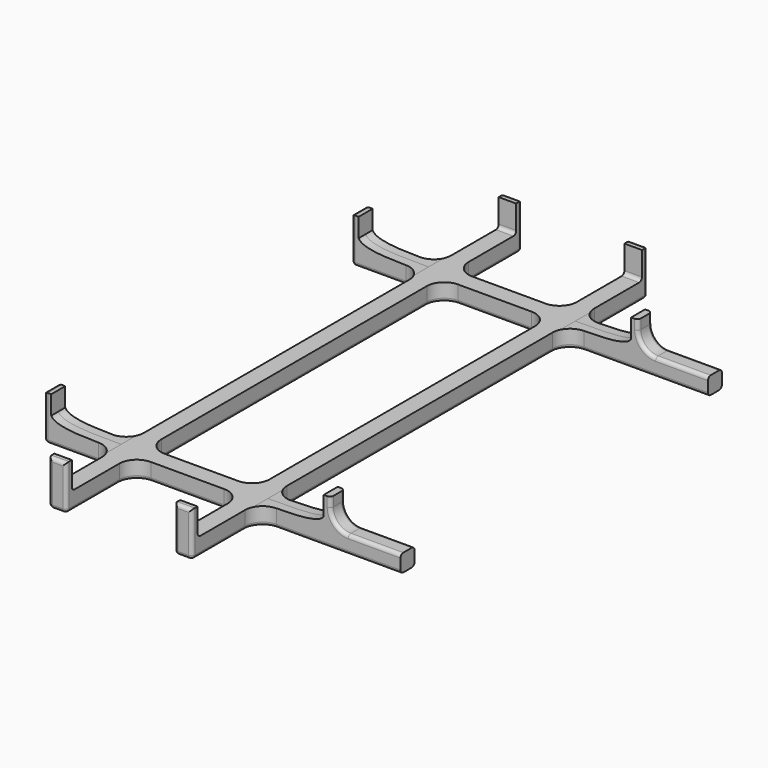
from build123d import *

# Parameters (mm, degrees)
F1_DEPTH  = 2.5
F3_DEPTH  = 2.5
F9_W      = 5
F9_H      = 5
F10_DEPTH = 20
F11_W     = 5
F11_H     = 5
F12_DEPTH = 20
F13_R     = 5
F14_R     = 1


with BuildPart() as f1:
    # F0 (on Front) → F1 (new body, symmetric)
    with BuildSketch(Plane.XZ):
        Polygon((-39, 7.8), (-41, 7.8), (-41, -5), (41, -5), (41, 7.8), (39, 7.8), (39, 2.4), (39, 0), (21, 0), (-21, 0), (-39, 0), (-39, 2.4), align=None)
        with BuildLine():
            Line((-39, 0), (-21, 0))
            add(Edge.make_bspline(
                [(-39, 2.4), (-37.8, 0), (-30, 0), (-21, 0)],
                knots=[0, 0, 0, 0, 18.1592951405, 18.1592951405, 18.1592951405, 18.1592951405], degree=3))
            Line((-39, 2.4), (-39, 0))
        make_face()
        with BuildLine():
            add(Edge.make_bspline(
                [(39, 2.4), (37.8, 0), (30, 0), (21, 0)],
                knots=[0, 0, 0, 0, 18.1592951405, 18.1592951405, 18.1592951405, 18.1592951405], degree=3))
            Line((21, 0), (39, 0))
            Line((39, 0), (39, 2.4))
        make_face()
    extrude(amount=F1_DEPTH, both=True)


with BuildPart() as f3:
    # F2 (on Right) → F3 (new body, symmetric)
    with BuildSketch(Plane.YZ):
        Polygon((-79.5, 7.8), (-81.5, 7.8), (-81.5, -5), (81.5, -5), (81.5, 7.8), (79.5, 7.8), (79.5, 0), (-79.5, 0), align=None)
    extrude(amount=F3_DEPTH, both=True)


with BuildPart() as f1_1:
    # F4: moved
    add(f1.part.moved(Location((0, -55, 0))))


with BuildPart() as f5_1:
    # F5: copy of F1
    add(f1_1.part.moved(Location((0, 110, 0))))


with BuildPart() as f3_1:
    # F6: moved
    add(f3.part.moved(Location((-18, 0, 0))))


with BuildPart() as f7_1:
    # F7: copy of F3
    add(f3_1.part.moved(Location((36, 0, 0))))


with BuildPart() as f1_2:
    add(f1_1.part)

    # F8: union F3, F7_1, F5_1
    add(f3_1.part)
    add(f7_1.part)
    add(f5_1.part)

    # F9 (on face) → F10 (join)
    with BuildSketch(Plane.YZ.offset(41)):
        with Locations((-55, -2.5)):
            Rectangle(F9_W, F9_H)
    extrude(amount=F10_DEPTH)

    # F11 (on face) → F12 (join)
    with BuildSketch(Plane.YZ.offset(41)):
        with Locations((55, -2.5)):
            Rectangle(F11_W, F11_H)
    extrude(amount=F12_DEPTH)

    # F13
    f13_edges = [f1_2.edges().sort_by_distance(p)[0] for p in [
        (-15.5, 52.5, -2.5),
        (-15.5, 57.5, -2.5),
        (-20.5, 52.5, -2.5),
        (-20.5, 57.5, -2.5),
        (15.5, 57.5, -2.5),
        (15.5, 52.5, -2.5),
        (20.5, 57.5, -2.5),
        (20.5, 52.5, -2.5),
        (20.5, -57.5, -2.5),
        (20.5, -52.5, -2.5),
        (15.5, -52.5, -2.5),
        (15.5, -57.5, -2.5),
        (-20.5, -57.5, -2.5),
        (-15.5, -57.5, -2.5),
        (-15.5, -52.5, -2.5),
        (-20.5, -52.5, -2.5),
        (41, -55, 0),
        (41, 55, 0),
    ]]
    fillet(f13_edges, radius=F13_R)

    # F14
    f14_edges = [f1_2.edges().sort_by_distance(p)[0] for p in [
        (53.5, 52.5, 0),
        (53.5, 57.5, 0),
        (53.5, -57.5, 0),
        (53.5, -52.5, 0),
        (43.25, -57.5, -5),
        (43.25, -52.5, -5),
        (43.25, 57.5, -5),
        (18, 81.5, -5),
        (15.5, 72, -5),
        (-18, 81.5, -5),
        (-20.5, 72, -5),
        (-41, 55, -5),
        (-33.25, 52.5, -5),
        (-41, -55, -5),
        (-33.25, -57.5, -5),
        (-18, -81.5, -5),
        (-15.5, -72, -5),
        (18, -81.5, -5),
        (-15.5, 0, -5),
        (18, -81.5, 7.8),
        (-18, -81.5, 7.8),
        (-20.5, -81.5, 1.4),
        (-15.5, -81.5, 1.4),
        (15.5, -81.5, 1.4),
        (20.5, -81.5, 1.4),
        (-41, -57.5, 1.4),
        (-41, -52.5, 1.4),
        (-41, -55, 7.8),
        (-41, 52.5, 1.4),
        (-41, 55, 7.8),
        (-41, 57.5, 1.4),
        (-20.5, 81.5, 1.4),
        (-18, 81.5, 7.8),
        (-15.5, 81.5, 1.4),
        (15.5, 81.5, 1.4),
        (18, 81.5, 7.8),
        (20.5, 81.5, 1.4),
        (18, 79.5, 0),
        (-18, 79.5, 0),
        (18, -79.5, 0),
        (-18, -79.5, 0),
        (-21.964466, -58.964466, -5),
        (-20.5, -72, -5),
        (-14.035534, -58.964466, -5),
        (-21.964466, -51.035534, -5),
        (0, -57.5, -5),
        (-20.5, 0, -5),
        (14.035534, -58.964466, -5),
        (-21.964466, 51.035534, -5),
        (15.5, -72, -5),
        (20.5, -72, -5),
        (-21.964466, 58.964466, -5),
        (21.964466, -58.964466, -5),
        (-15.5, 72, -5),
        (21.964466, -51.035534, -5),
        (-14.035534, 58.964466, -5),
        (20.5, 0, -5),
        (0, 57.5, -5),
        (21.964466, 51.035534, -5),
        (14.035534, 58.964466, -5),
        (21.964466, 58.964466, -5),
        (20.5, 72, -5),
        (0, -52.5, -5),
        (14.035534, -51.035534, -5),
        (-14.035534, -51.035534, -5),
        (15.5, 0, -5),
        (14.035534, 51.035534, -5),
        (-14.035534, 51.035534, -5),
        (0, 52.5, -5),
        (-33.25, -52.5, -5),
        (-33.25, 57.5, -5),
        (43.25, 52.5, -5),
        (42.464466, -57.5, 1.464466),
        (41, -57.5, 6.4),
        (42.464466, -52.5, 1.464466),
        (41, -52.5, 6.4),
        (42.464466, 52.5, 1.464466),
        (41, 52.5, 6.4),
        (42.464466, 57.5, 1.464466),
        (41, 57.5, 6.4),
    ]]
    fillet(f14_edges, radius=F14_R)


solid = f1_2.part
